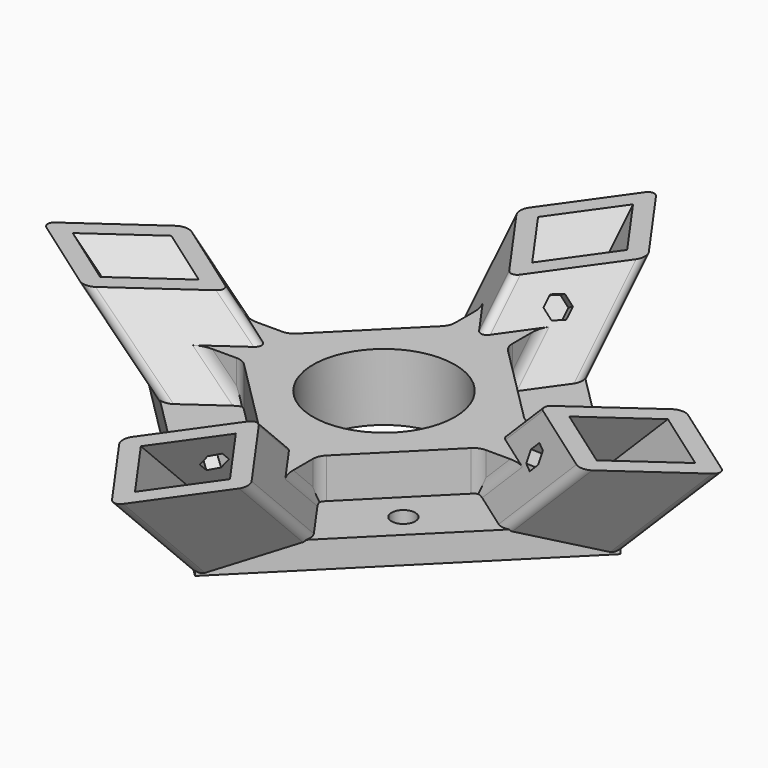
from build123d import *

# Parameters (mm, degrees)
F1_DEPTH      = 4.318
F9_DEPTH      = 2.54
F10_COUNT     = 4
F10_ANGLE     = 270
F14_DEPTH     = 10.795
F12_R         = 11.43
F15_DEPTH     = 25.4
F16_R         = 1.905
F17_DEPTH     = 25.4
F25_W         = 111.76
F25_H         = 15.24
F26_DEPTH     = 152.4
F27_T4_DEPTH  = 14.9351248517
F27_T9_DEPTH  = 24.0949860952
F27_T14_DEPTH = 24.0949860952
F27_T19_DEPTH = 30.2015602576
F27_T24_DEPTH = 30.2015602576
F27_T29_DEPTH = 24.0949860952
F27_T34_DEPTH = 24.0949860952
F27_T39_DEPTH = 24.0949860952
F27_T44_DEPTH = 24.0949860952
F27_T49_DEPTH = 30.2015602576
F27_T54_DEPTH = 30.2015602576
F27_T59_DEPTH = 24.0949860952
F27_T64_DEPTH = 24.0949860952
F27_T69_DEPTH = 14.9351248517
F28_T4_DEPTH  = 24.0949860952
F28_T9_DEPTH  = 24.0949860952
F28_T14_DEPTH = 30.2015602576
F28_T19_DEPTH = 30.2015602576
F28_T24_DEPTH = 24.0949860952
F28_T29_DEPTH = 24.0949860952
F28_T34_DEPTH = 14.9351248517
F28_T39_DEPTH = 14.9351248517
F28_T44_DEPTH = 24.0949860952
F28_T49_DEPTH = 24.0949860952
F28_T54_DEPTH = 24.0949860952
F28_T59_DEPTH = 24.0949860952
F28_T64_DEPTH = 30.2015602576
F28_T69_DEPTH = 30.2015602576
F29_T1_DEPTH  = 9.1072561211
F29_T6_DEPTH  = 14.4203734856
F29_T11_DEPTH = 14.4203734854
F29_T16_DEPTH = 14.4203734856
F29_T21_DEPTH = 14.4203734854
F29_T26_DEPTH = 14.4203734856
F29_T31_DEPTH = 14.4203734854
F29_T36_DEPTH = 14.4203734854
F29_T41_DEPTH = 14.4203734856


# Not quite as in the source:
# - a fillet or chamfer that OpenCascade refuses, or shapes differently, is made with other operations: its cross-section is extruded or revolved along the edge and cut away or added


with BuildPart() as f1:
    # F0 (on Top) → F1 (new body)
    with BuildSketch(Plane.XY):
        Polygon((38.1, 0), (0, 38.1), (-38.1, 0), (0, -38.1), align=None)
    extrude(amount=F1_DEPTH)

    # F5 (on offset) → F6 (join, up to the next surface of F1)
    with BuildSketch(Plane(origin=(0, -35.9210244843, 35.9210244843), x_dir=(1, 0, 0), z_dir=(0, 0.7071067812, -0.7071067812))):
        Polygon((10.5607811984, 16.3799871648), (0, 26.9407683632), (-10.5607811984, 16.3799871648), (0, 5.8192059665), align=None)
        Polygon((-7.1842048969, 16.3799871648), (0, 23.5641920617), (7.1842048969, 16.3799871648), (0, 9.195782268), align=None, mode=Mode.SUBTRACT)
    extrude(until=Until.NEXT)

    # F8 (on offset) → F9 (cut)
    with BuildSketch(Plane(origin=(2.9096029833, -2.0574, -2.0574), x_dir=(-0.4082482905, -0.8660254038, 0.2886751346), z_dir=(-0.7071067812, 0.5, 0.5))):
        Polygon((30.7118833173, 5.5090421757), (32.268461045, 6.6097088424), (32.0935446144, 8.5080780308), (30.3620504561, 9.3057805526), (28.8054727285, 8.2051138859), (28.9803891591, 6.3067446975), align=None)
    extrude(amount=-F9_DEPTH, mode=Mode.SUBTRACT)


with BuildPart() as f10_1:
    # F10: instance of F1
    add(f1.part.rotate(Axis((0, 0, 13.9133725866), (0, 0, 1)), 1 * F10_ANGLE / (F10_COUNT - 1)))


with BuildPart() as f10_2:
    # F10: instance of F1
    add(f1.part.rotate(Axis((0, 0, 13.9133725866), (0, 0, 1)), 2 * F10_ANGLE / (F10_COUNT - 1)))


with BuildPart() as f10_3:
    # F10: instance of F1
    add(f1.part.rotate(Axis((0, 0, 13.9133725866), (0, 0, 1)), 3 * F10_ANGLE / (F10_COUNT - 1)))


with BuildPart() as f1_1:
    add(f1.part)

    add(f10_1.part)  # F14 merges F10_1

    add(f10_2.part)  # F14 merges F10_2

    add(f10_3.part)  # F14 merges F10_3
    # F13 (on Top) → F14 (join)
    with BuildSketch(Plane.XY):
        Polygon((19.05, 4.597891134), (4.5978911339, 19.05), (-4.5978911339, 19.05), (-19.05, 4.5978911339), (-19.05, -4.597891134), (-4.5978911339, -19.05), (4.597891134, -19.05), (19.05, -4.5978911339), align=None)
    extrude(amount=F14_DEPTH)

    # F12 (on offset) → F15 (cut)
    with BuildSketch(Plane.XY.offset(25.4)):
        Circle(F12_R)
    extrude(amount=-F15_DEPTH, mode=Mode.SUBTRACT)

    # F16 (on offset) → F17 (cut)
    with BuildSketch(Plane.XY.offset(25.4)):
        with Locations((-15.6256456507, 15.6256456507)):
            Circle(F16_R)
        with Locations((15.6256456507, 15.6256456507)):
            Circle(F16_R)
        with Locations((15.6256456507, -15.6256456507)):
            Circle(F16_R)
        with Locations((-15.6256456507, -15.6256456507)):
            Circle(F16_R)
    extrude(amount=-F17_DEPTH, mode=Mode.SUBTRACT)

    # F18: union 

    # F19: union 

    # F19_face (on face) → F20 (join, up to the next surface of F1)
    with BuildSketch(Plane(origin=(-19.05, 3.0712475933, 8.6360000001), x_dir=(0, -1, 0), z_dir=(-1, 0, 0))):
        Polygon((3.0532870811, 2.1589999999), (-1.5266435405, 2.1589999999), (-1.5266435405, -4.3180000001), align=None)
        Polygon((7.6691387273, -4.3180000001), (7.6691387273, 2.1589999999), (3.0892081056, 2.1589999999), align=None)
    extrude(until=Until.NEXT)

    # F18_face (on face) → F21 (join, up to the next surface of F1)
    with BuildSketch(Plane(origin=(-3.0712475934, 19.05, 8.636), x_dir=(-1, 0, 0), z_dir=(0, 1, 0))):
        Polygon((1.5266435406, -4.318), (1.5266435406, 2.159), (-3.0532870811, 2.159), align=None)
        Polygon((-3.0892081056, 2.159), (-7.6691387273, 2.159), (-7.6691387273, -4.318), align=None)
    extrude(until=Until.NEXT)

    # F19_face1 (on face) → F22 (join, up to the next surface of F1)
    with BuildSketch(Plane(origin=(19.05, -3.0712475933, 8.6360000001), x_dir=(0, 1, 0), z_dir=(1, 0, 0))):
        Polygon((3.0532870811, 2.1589999999), (-1.5266435405, 2.1589999999), (-1.5266435405, -4.3180000001), align=None)
        Polygon((7.6691387273, -4.3180000001), (7.6691387273, 2.1589999999), (3.0892081056, 2.1589999999), align=None)
    extrude(until=Until.NEXT)

    # F19_face2 (on face) → F23 (join, up to the next surface of F1)
    with BuildSketch(Plane(origin=(3.0712475934, -19.05, 8.636), x_dir=(1, 0, 0), z_dir=(0, -1, 0))):
        Polygon((1.5266435406, -4.318), (1.5266435406, 2.159), (-3.0532870811, 2.159), align=None)
        Polygon((-7.6691387273, -4.3179999998), (-3.0892081056, 2.159), (-7.6691387273, 2.159), align=None)
    extrude(until=Until.NEXT)

    # F25 (on offset) → F26 (cut)
    with BuildSketch(Plane.YZ.offset(63.5)):
        with Locations((0, 24.4856)):
            Rectangle(F25_W, F25_H)
    extrude(amount=-F26_DEPTH, mode=Mode.SUBTRACT)

    # F27: fillet of radius 1.27 on 8 edges, made by hand


with BuildPart() as f27_tool2:
    # F27_s3 → F27_t4 (new body)
    with BuildSketch(Plane(origin=(0, 23.2254640303, 23.2254640303), x_dir=(1, 0, 0), z_dir=(0, -0.7071067812, -0.7071067812))):
        with BuildLine():
            ThreePointArc((0.8980256121, -6.7172315786), (0, -6.3452571907), (-0.8980256121, -6.7172315786))
            Line((-0.8980256121, -6.7172315786), (0, -5.8192059665))
            Line((0, -5.8192059665), (0.8980256121, -6.7172315786))
        make_face()
    extrude(amount=F27_T4_DEPTH)

    split(bisect_by=Plane.XY.offset(10.795), keep=Keep.TOP)


with BuildPart() as f1_2:
    add(f1_1.part)

    # F27_t1: cut F27_tool2
    add(f27_tool2.part, mode=Mode.SUBTRACT)


with BuildPart() as f27_tool7:
    # F27_s8 → F27_t9 (new body)
    with BuildSketch(Plane(origin=(0, 30.6930640303, 30.6930640303), x_dir=(1, 0, 0), z_dir=(0, -0.7071067812, -0.7071067812))):
        with BuildLine():
            ThreePointArc((9.6627555863, -17.2780127769), (10.0347299742, -16.3799871648), (9.6627555863, -15.4819615527))
            Line((9.6627555863, -15.4819615527), (10.5607811984, -16.3799871648))
            Line((10.5607811984, -16.3799871648), (9.6627555863, -17.2780127769))
        make_face()
    extrude(amount=F27_T9_DEPTH)

    split(bisect_by=Plane.XY.offset(4.318), keep=Keep.TOP)


with BuildPart() as f1_3:
    add(f1_2.part)

    # F27_t6: cut F27_tool7
    add(f27_tool7.part, mode=Mode.SUBTRACT)


with BuildPart() as f27_tool12:
    # F27_s13 → F27_t14 (new body)
    with BuildSketch(Plane(origin=(0, 30.6930640303, 30.6930640303), x_dir=(1, 0, 0), z_dir=(0, -0.7071067812, -0.7071067812))):
        with BuildLine():
            ThreePointArc((9.6627555863, -17.2780127769), (10.0347299742, -16.3799871648), (9.6627555863, -15.4819615527))
            Line((9.6627555863, -15.4819615527), (10.5607811984, -16.3799871648))
            Line((10.5607811984, -16.3799871648), (9.6627555863, -17.2780127769))
        make_face()
    extrude(amount=F27_T14_DEPTH)

    split(bisect_by=Plane(origin=(19.05, 19.05, 0), x_dir=(0, 0, 1), z_dir=(0.7071067812, 0.7071067812, 0)), keep=Keep.TOP)


with BuildPart() as f1_4:
    add(f1_3.part)

    # F27_t11: cut F27_tool12
    add(f27_tool12.part, mode=Mode.SUBTRACT)


with BuildPart() as f27_tool17:
    # F27_s18 → F27_t19 (new body)
    with BuildSketch(Plane(origin=(0, 38.1606640303, 38.1606640303), x_dir=(1, 0, 0), z_dir=(0, -0.7071067812, -0.7071067812))):
        with BuildLine():
            ThreePointArc((0.8980256121, -26.0427427511), (0, -26.414717139), (-0.8980256121, -26.0427427511))
            Line((-0.8980256121, -26.0427427511), (0, -26.9407683632))
            Line((0, -26.9407683632), (0.8980256121, -26.0427427511))
        make_face()
    extrude(amount=F27_T19_DEPTH)

    split(bisect_by=Plane(origin=(-19.05, 19.05, 0), x_dir=(0, 0, 1), z_dir=(-0.7071067812, 0.7071067812, 0)), keep=Keep.TOP)


with BuildPart() as f1_5:
    add(f1_4.part)

    # F27_t16: cut F27_tool17
    add(f27_tool17.part, mode=Mode.SUBTRACT)


with BuildPart() as f27_tool22:
    # F27_s23 → F27_t24 (new body)
    with BuildSketch(Plane(origin=(0, 38.1606640303, 38.1606640303), x_dir=(1, 0, 0), z_dir=(0, -0.7071067812, -0.7071067812))):
        with BuildLine():
            ThreePointArc((0.8980256121, -26.0427427511), (0, -26.414717139), (-0.8980256121, -26.0427427511))
            Line((-0.8980256121, -26.0427427511), (0, -26.9407683632))
            Line((0, -26.9407683632), (0.8980256121, -26.0427427511))
        make_face()
    extrude(amount=F27_T24_DEPTH)

    split(bisect_by=Plane(origin=(19.05, 19.05, 0), x_dir=(0, 0, 1), z_dir=(0.7071067812, 0.7071067812, 0)), keep=Keep.TOP)


with BuildPart() as f1_6:
    add(f1_5.part)

    # F27_t21: cut F27_tool22
    add(f27_tool22.part, mode=Mode.SUBTRACT)


with BuildPart() as f27_tool27:
    # F27_s28 → F27_t29 (new body)
    with BuildSketch(Plane(origin=(0, 30.6930640303, 30.6930640303), x_dir=(1, 0, 0), z_dir=(0, -0.7071067812, -0.7071067812))):
        with BuildLine():
            ThreePointArc((-9.6627555863, -17.2780127769), (-10.0347299742, -16.3799871648), (-9.6627555863, -15.4819615527))
            Line((-9.6627555863, -15.4819615527), (-10.5607811984, -16.3799871648))
            Line((-10.5607811984, -16.3799871648), (-9.6627555863, -17.2780127769))
        make_face()
    extrude(amount=F27_T29_DEPTH)

    split(bisect_by=Plane.XY.offset(4.318), keep=Keep.TOP)


with BuildPart() as f1_7:
    add(f1_6.part)

    # F27_t26: cut F27_tool27
    add(f27_tool27.part, mode=Mode.SUBTRACT)


with BuildPart() as f27_tool32:
    # F27_s33 → F27_t34 (new body)
    with BuildSketch(Plane(origin=(0, 30.6930640303, 30.6930640303), x_dir=(1, 0, 0), z_dir=(0, -0.7071067812, -0.7071067812))):
        with BuildLine():
            ThreePointArc((-9.6627555863, -17.2780127769), (-10.0347299742, -16.3799871648), (-9.6627555863, -15.4819615527))
            Line((-9.6627555863, -15.4819615527), (-10.5607811984, -16.3799871648))
            Line((-10.5607811984, -16.3799871648), (-9.6627555863, -17.2780127769))
        make_face()
    extrude(amount=F27_T34_DEPTH)

    split(bisect_by=Plane(origin=(-19.05, 19.05, 0), x_dir=(0, 0, 1), z_dir=(-0.7071067812, 0.7071067812, 0)), keep=Keep.TOP)


with BuildPart() as f1_8:
    add(f1_7.part)

    # F27_t31: cut F27_tool32
    add(f27_tool32.part, mode=Mode.SUBTRACT)


with BuildPart() as f27_tool37:
    # F27_s38 → F27_t39 (new body)
    with BuildSketch(Plane(origin=(30.6930640303, 0, 30.6930640303), x_dir=(0, 1, 0), z_dir=(-0.7071067812, 0, -0.7071067812))):
        with BuildLine():
            ThreePointArc((9.6627555863, 17.2780127769), (10.0347299742, 16.3799871648), (9.6627555863, 15.4819615527))
            Line((9.6627555863, 15.4819615527), (10.5607811984, 16.3799871648))
            Line((10.5607811984, 16.3799871648), (9.6627555863, 17.2780127769))
        make_face()
    extrude(amount=F27_T39_DEPTH)

    split(bisect_by=Plane.XY.offset(4.318), keep=Keep.TOP)


with BuildPart() as f1_9:
    add(f1_8.part)

    # F27_t36: cut F27_tool37
    add(f27_tool37.part, mode=Mode.SUBTRACT)


with BuildPart() as f27_tool42:
    # F27_s43 → F27_t44 (new body)
    with BuildSketch(Plane(origin=(30.6930640303, 0, 30.6930640303), x_dir=(0, 1, 0), z_dir=(-0.7071067812, 0, -0.7071067812))):
        with BuildLine():
            ThreePointArc((9.6627555863, 17.2780127769), (10.0347299742, 16.3799871648), (9.6627555863, 15.4819615527))
            Line((9.6627555863, 15.4819615527), (10.5607811984, 16.3799871648))
            Line((10.5607811984, 16.3799871648), (9.6627555863, 17.2780127769))
        make_face()
    extrude(amount=F27_T44_DEPTH)

    split(bisect_by=Plane(origin=(19.05, 19.05, 0), x_dir=(0, 0, 1), z_dir=(0.7071067812, 0.7071067812, 0)), keep=Keep.TOP)


with BuildPart() as f1_10:
    add(f1_9.part)

    # F27_t41: cut F27_tool42
    add(f27_tool42.part, mode=Mode.SUBTRACT)


with BuildPart() as f27_tool47:
    # F27_s48 → F27_t49 (new body)
    with BuildSketch(Plane(origin=(38.1606640303, 0, 38.1606640303), x_dir=(0, 1, 0), z_dir=(-0.7071067812, 0, -0.7071067812))):
        with BuildLine():
            ThreePointArc((-0.8980256121, 26.0427427511), (0, 26.414717139), (0.8980256121, 26.0427427511))
            Line((0.8980256121, 26.0427427511), (0, 26.9407683632))
            Line((0, 26.9407683632), (-0.8980256121, 26.0427427511))
        make_face()
    extrude(amount=F27_T49_DEPTH)

    split(bisect_by=Plane(origin=(19.05, 19.05, 0), x_dir=(0, 0, 1), z_dir=(0.7071067812, 0.7071067812, 0)), keep=Keep.TOP)


with BuildPart() as f1_11:
    add(f1_10.part)

    # F27_t46: cut F27_tool47
    add(f27_tool47.part, mode=Mode.SUBTRACT)


with BuildPart() as f27_tool52:
    # F27_s53 → F27_t54 (new body)
    with BuildSketch(Plane(origin=(38.1606640303, 0, 38.1606640303), x_dir=(0, 1, 0), z_dir=(-0.7071067812, 0, -0.7071067812))):
        with BuildLine():
            ThreePointArc((-0.8980256121, 26.0427427511), (0, 26.414717139), (0.8980256121, 26.0427427511))
            Line((0.8980256121, 26.0427427511), (0, 26.9407683632))
            Line((0, 26.9407683632), (-0.8980256121, 26.0427427511))
        make_face()
    extrude(amount=F27_T54_DEPTH)

    split(bisect_by=Plane(origin=(19.05, -19.05, 0), x_dir=(0, 0, 1), z_dir=(0.7071067812, -0.7071067812, 0)), keep=Keep.TOP)


with BuildPart() as f1_12:
    add(f1_11.part)

    # F27_t51: cut F27_tool52
    add(f27_tool52.part, mode=Mode.SUBTRACT)


with BuildPart() as f27_tool57:
    # F27_s58 → F27_t59 (new body)
    with BuildSketch(Plane(origin=(30.6930640303, 0, 30.6930640303), x_dir=(0, 1, 0), z_dir=(-0.7071067812, 0, -0.7071067812))):
        with BuildLine():
            ThreePointArc((-9.6627555863, 17.2780127769), (-10.0347299742, 16.3799871648), (-9.6627555863, 15.4819615527))
            Line((-9.6627555863, 15.4819615527), (-10.5607811984, 16.3799871648))
            Line((-10.5607811984, 16.3799871648), (-9.6627555863, 17.2780127769))
        make_face()
    extrude(amount=F27_T59_DEPTH)

    split(bisect_by=Plane.XY.offset(4.318), keep=Keep.TOP)


with BuildPart() as f1_13:
    add(f1_12.part)

    # F27_t56: cut F27_tool57
    add(f27_tool57.part, mode=Mode.SUBTRACT)


with BuildPart() as f27_tool62:
    # F27_s63 → F27_t64 (new body)
    with BuildSketch(Plane(origin=(30.6930640303, 0, 30.6930640303), x_dir=(0, 1, 0), z_dir=(-0.7071067812, 0, -0.7071067812))):
        with BuildLine():
            ThreePointArc((-9.6627555863, 17.2780127769), (-10.0347299742, 16.3799871648), (-9.6627555863, 15.4819615527))
            Line((-9.6627555863, 15.4819615527), (-10.5607811984, 16.3799871648))
            Line((-10.5607811984, 16.3799871648), (-9.6627555863, 17.2780127769))
        make_face()
    extrude(amount=F27_T64_DEPTH)

    split(bisect_by=Plane(origin=(19.05, -19.05, 0), x_dir=(0, 0, 1), z_dir=(0.7071067812, -0.7071067812, 0)), keep=Keep.TOP)


with BuildPart() as f1_14:
    add(f1_13.part)

    # F27_t61: cut F27_tool62
    add(f27_tool62.part, mode=Mode.SUBTRACT)


with BuildPart() as f27_tool67:
    # F27_s68 → F27_t69 (new body)
    with BuildSketch(Plane(origin=(23.2254640303, 0, 23.2254640303), x_dir=(0, 1, 0), z_dir=(-0.7071067812, 0, -0.7071067812))):
        with BuildLine():
            ThreePointArc((-0.8980256121, 6.7172315786), (0, 6.3452571907), (0.8980256121, 6.7172315786))
            Line((0.8980256121, 6.7172315786), (0, 5.8192059665))
            Line((0, 5.8192059665), (-0.8980256121, 6.7172315786))
        make_face()
    extrude(amount=F27_T69_DEPTH)

    split(bisect_by=Plane.XY.offset(10.795), keep=Keep.TOP)


with BuildPart() as f1_15:
    add(f1_14.part)

    # F27_t66: cut F27_tool67
    add(f27_tool67.part, mode=Mode.SUBTRACT)

    # F28: fillet of radius 1.27 on 8 edges, made by hand


with BuildPart() as f28_tool2:
    # F28_s3 → F28_t4 (new body)
    with BuildSketch(Plane(origin=(0, -30.6930640303, 30.6930640303), x_dir=(1, 0, 0), z_dir=(0, 0.7071067812, -0.7071067812))):
        with BuildLine():
            ThreePointArc((-9.6627555863, 17.2780127769), (-10.0347299742, 16.3799871648), (-9.6627555863, 15.4819615527))
            Line((-9.6627555863, 15.4819615527), (-10.5607811984, 16.3799871648))
            Line((-10.5607811984, 16.3799871648), (-9.6627555863, 17.2780127769))
        make_face()
    extrude(amount=F28_T4_DEPTH)

    split(bisect_by=Plane.XY.offset(4.318), keep=Keep.TOP)


with BuildPart() as f1_16:
    add(f1_15.part)

    # F28_t1: cut F28_tool2
    add(f28_tool2.part, mode=Mode.SUBTRACT)


with BuildPart() as f28_tool7:
    # F28_s8 → F28_t9 (new body)
    with BuildSketch(Plane(origin=(0, -30.6930640303, 30.6930640303), x_dir=(1, 0, 0), z_dir=(0, 0.7071067812, -0.7071067812))):
        with BuildLine():
            ThreePointArc((-9.6627555863, 17.2780127769), (-10.0347299742, 16.3799871648), (-9.6627555863, 15.4819615527))
            Line((-9.6627555863, 15.4819615527), (-10.5607811984, 16.3799871648))
            Line((-10.5607811984, 16.3799871648), (-9.6627555863, 17.2780127769))
        make_face()
    extrude(amount=F28_T9_DEPTH)

    split(bisect_by=Plane(origin=(-19.05, -19.05, 0), x_dir=(0, 0, 1), z_dir=(-0.7071067812, -0.7071067812, 0)), keep=Keep.TOP)


with BuildPart() as f1_17:
    add(f1_16.part)

    # F28_t6: cut F28_tool7
    add(f28_tool7.part, mode=Mode.SUBTRACT)


with BuildPart() as f28_tool12:
    # F28_s13 → F28_t14 (new body)
    with BuildSketch(Plane(origin=(0, -38.1606640303, 38.1606640303), x_dir=(1, 0, 0), z_dir=(0, 0.7071067812, -0.7071067812))):
        with BuildLine():
            ThreePointArc((0.8980256121, 26.0427427511), (0, 26.414717139), (-0.8980256121, 26.0427427511))
            Line((-0.8980256121, 26.0427427511), (0, 26.9407683632))
            Line((0, 26.9407683632), (0.8980256121, 26.0427427511))
        make_face()
    extrude(amount=F28_T14_DEPTH)

    split(bisect_by=Plane(origin=(-19.05, -19.05, 0), x_dir=(0, 0, 1), z_dir=(-0.7071067812, -0.7071067812, 0)), keep=Keep.TOP)


with BuildPart() as f1_18:
    add(f1_17.part)

    # F28_t11: cut F28_tool12
    add(f28_tool12.part, mode=Mode.SUBTRACT)


with BuildPart() as f28_tool17:
    # F28_s18 → F28_t19 (new body)
    with BuildSketch(Plane(origin=(0, -38.1606640303, 38.1606640303), x_dir=(1, 0, 0), z_dir=(0, 0.7071067812, -0.7071067812))):
        with BuildLine():
            ThreePointArc((0.8980256121, 26.0427427511), (0, 26.414717139), (-0.8980256121, 26.0427427511))
            Line((-0.8980256121, 26.0427427511), (0, 26.9407683632))
            Line((0, 26.9407683632), (0.8980256121, 26.0427427511))
        make_face()
    extrude(amount=F28_T19_DEPTH)

    split(bisect_by=Plane(origin=(19.05, -19.05, 0), x_dir=(0, 0, 1), z_dir=(0.7071067812, -0.7071067812, 0)), keep=Keep.TOP)


with BuildPart() as f1_19:
    add(f1_18.part)

    # F28_t16: cut F28_tool17
    add(f28_tool17.part, mode=Mode.SUBTRACT)


with BuildPart() as f28_tool22:
    # F28_s23 → F28_t24 (new body)
    with BuildSketch(Plane(origin=(0, -30.6930640303, 30.6930640303), x_dir=(1, 0, 0), z_dir=(0, 0.7071067812, -0.7071067812))):
        with BuildLine():
            ThreePointArc((9.6627555863, 17.2780127769), (10.0347299742, 16.3799871648), (9.6627555863, 15.4819615527))
            Line((9.6627555863, 15.4819615527), (10.5607811984, 16.3799871648))
            Line((10.5607811984, 16.3799871648), (9.6627555863, 17.2780127769))
        make_face()
    extrude(amount=F28_T24_DEPTH)

    split(bisect_by=Plane.XY.offset(4.318), keep=Keep.TOP)


with BuildPart() as f1_20:
    add(f1_19.part)

    # F28_t21: cut F28_tool22
    add(f28_tool22.part, mode=Mode.SUBTRACT)


with BuildPart() as f28_tool27:
    # F28_s28 → F28_t29 (new body)
    with BuildSketch(Plane(origin=(0, -30.6930640303, 30.6930640303), x_dir=(1, 0, 0), z_dir=(0, 0.7071067812, -0.7071067812))):
        with BuildLine():
            ThreePointArc((9.6627555863, 17.2780127769), (10.0347299742, 16.3799871648), (9.6627555863, 15.4819615527))
            Line((9.6627555863, 15.4819615527), (10.5607811984, 16.3799871648))
            Line((10.5607811984, 16.3799871648), (9.6627555863, 17.2780127769))
        make_face()
    extrude(amount=F28_T29_DEPTH)

    split(bisect_by=Plane(origin=(19.05, -19.05, 0), x_dir=(0, 0, 1), z_dir=(0.7071067812, -0.7071067812, 0)), keep=Keep.TOP)


with BuildPart() as f1_21:
    add(f1_20.part)

    # F28_t26: cut F28_tool27
    add(f28_tool27.part, mode=Mode.SUBTRACT)


with BuildPart() as f28_tool32:
    # F28_s33 → F28_t34 (new body)
    with BuildSketch(Plane(origin=(0, -23.2254640303, 23.2254640303), x_dir=(1, 0, 0), z_dir=(0, 0.7071067812, -0.7071067812))):
        with BuildLine():
            ThreePointArc((0.8980256121, 6.7172315786), (0, 6.3452571907), (-0.8980256121, 6.7172315786))
            Line((-0.8980256121, 6.7172315786), (0, 5.8192059665))
            Line((0, 5.8192059665), (0.8980256121, 6.7172315786))
        make_face()
    extrude(amount=F28_T34_DEPTH)

    split(bisect_by=Plane.XY.offset(10.795), keep=Keep.TOP)


with BuildPart() as f1_22:
    add(f1_21.part)

    # F28_t31: cut F28_tool32
    add(f28_tool32.part, mode=Mode.SUBTRACT)


with BuildPart() as f28_tool37:
    # F28_s38 → F28_t39 (new body)
    with BuildSketch(Plane(origin=(-23.2254640303, 0, 23.2254640303), x_dir=(0, 1, 0), z_dir=(0.7071067812, 0, -0.7071067812))):
        with BuildLine():
            ThreePointArc((-0.8980256121, -6.7172315786), (0, -6.3452571907), (0.8980256121, -6.7172315786))
            Line((0.8980256121, -6.7172315786), (0, -5.8192059665))
            Line((0, -5.8192059665), (-0.8980256121, -6.7172315786))
        make_face()
    extrude(amount=F28_T39_DEPTH)

    split(bisect_by=Plane.XY.offset(10.795), keep=Keep.TOP)


with BuildPart() as f1_23:
    add(f1_22.part)

    # F28_t36: cut F28_tool37
    add(f28_tool37.part, mode=Mode.SUBTRACT)


with BuildPart() as f28_tool42:
    # F28_s43 → F28_t44 (new body)
    with BuildSketch(Plane(origin=(-30.6930640303, 0, 30.6930640303), x_dir=(0, 1, 0), z_dir=(0.7071067812, 0, -0.7071067812))):
        with BuildLine():
            ThreePointArc((-9.6627555863, -17.2780127769), (-10.0347299742, -16.3799871648), (-9.6627555863, -15.4819615527))
            Line((-9.6627555863, -15.4819615527), (-10.5607811984, -16.3799871648))
            Line((-10.5607811984, -16.3799871648), (-9.6627555863, -17.2780127769))
        make_face()
    extrude(amount=F28_T44_DEPTH)

    split(bisect_by=Plane.XY.offset(4.318), keep=Keep.TOP)


with BuildPart() as f1_24:
    add(f1_23.part)

    # F28_t41: cut F28_tool42
    add(f28_tool42.part, mode=Mode.SUBTRACT)


with BuildPart() as f28_tool47:
    # F28_s48 → F28_t49 (new body)
    with BuildSketch(Plane(origin=(-30.6930640303, 0, 30.6930640303), x_dir=(0, 1, 0), z_dir=(0.7071067812, 0, -0.7071067812))):
        with BuildLine():
            ThreePointArc((-9.6627555863, -17.2780127769), (-10.0347299742, -16.3799871648), (-9.6627555863, -15.4819615527))
            Line((-9.6627555863, -15.4819615527), (-10.5607811984, -16.3799871648))
            Line((-10.5607811984, -16.3799871648), (-9.6627555863, -17.2780127769))
        make_face()
    extrude(amount=F28_T49_DEPTH)

    split(bisect_by=Plane(origin=(-19.05, -19.05, 0), x_dir=(0, 0, 1), z_dir=(-0.7071067812, -0.7071067812, 0)), keep=Keep.TOP)


with BuildPart() as f1_25:
    add(f1_24.part)

    # F28_t46: cut F28_tool47
    add(f28_tool47.part, mode=Mode.SUBTRACT)


with BuildPart() as f28_tool52:
    # F28_s53 → F28_t54 (new body)
    with BuildSketch(Plane(origin=(-30.6930640303, 0, 30.6930640303), x_dir=(0, 1, 0), z_dir=(0.7071067812, 0, -0.7071067812))):
        with BuildLine():
            ThreePointArc((9.6627555863, -17.2780127769), (10.0347299742, -16.3799871648), (9.6627555863, -15.4819615527))
            Line((9.6627555863, -15.4819615527), (10.5607811984, -16.3799871648))
            Line((10.5607811984, -16.3799871648), (9.6627555863, -17.2780127769))
        make_face()
    extrude(amount=F28_T54_DEPTH)

    split(bisect_by=Plane.XY.offset(4.318), keep=Keep.TOP)


with BuildPart() as f1_26:
    add(f1_25.part)

    # F28_t51: cut F28_tool52
    add(f28_tool52.part, mode=Mode.SUBTRACT)


with BuildPart() as f28_tool57:
    # F28_s58 → F28_t59 (new body)
    with BuildSketch(Plane(origin=(-30.6930640303, 0, 30.6930640303), x_dir=(0, 1, 0), z_dir=(0.7071067812, 0, -0.7071067812))):
        with BuildLine():
            ThreePointArc((9.6627555863, -17.2780127769), (10.0347299742, -16.3799871648), (9.6627555863, -15.4819615527))
            Line((9.6627555863, -15.4819615527), (10.5607811984, -16.3799871648))
            Line((10.5607811984, -16.3799871648), (9.6627555863, -17.2780127769))
        make_face()
    extrude(amount=F28_T59_DEPTH)

    split(bisect_by=Plane(origin=(-19.05, 19.05, 0), x_dir=(0, 0, 1), z_dir=(-0.7071067812, 0.7071067812, 0)), keep=Keep.TOP)


with BuildPart() as f1_27:
    add(f1_26.part)

    # F28_t56: cut F28_tool57
    add(f28_tool57.part, mode=Mode.SUBTRACT)


with BuildPart() as f28_tool62:
    # F28_s63 → F28_t64 (new body)
    with BuildSketch(Plane(origin=(-38.1606640303, 0, 38.1606640303), x_dir=(0, 1, 0), z_dir=(0.7071067812, 0, -0.7071067812))):
        with BuildLine():
            ThreePointArc((-0.8980256121, -26.0427427511), (0, -26.414717139), (0.8980256121, -26.0427427511))
            Line((0.8980256121, -26.0427427511), (0, -26.9407683632))
            Line((0, -26.9407683632), (-0.8980256121, -26.0427427511))
        make_face()
    extrude(amount=F28_T64_DEPTH)

    split(bisect_by=Plane(origin=(-19.05, 19.05, 0), x_dir=(0, 0, 1), z_dir=(-0.7071067812, 0.7071067812, 0)), keep=Keep.TOP)


with BuildPart() as f1_28:
    add(f1_27.part)

    # F28_t61: cut F28_tool62
    add(f28_tool62.part, mode=Mode.SUBTRACT)


with BuildPart() as f28_tool67:
    # F28_s68 → F28_t69 (new body)
    with BuildSketch(Plane(origin=(-38.1606640303, 0, 38.1606640303), x_dir=(0, 1, 0), z_dir=(0.7071067812, 0, -0.7071067812))):
        with BuildLine():
            ThreePointArc((-0.8980256121, -26.0427427511), (0, -26.414717139), (0.8980256121, -26.0427427511))
            Line((0.8980256121, -26.0427427511), (0, -26.9407683632))
            Line((0, -26.9407683632), (-0.8980256121, -26.0427427511))
        make_face()
    extrude(amount=F28_T69_DEPTH)

    split(bisect_by=Plane(origin=(-19.05, -19.05, 0), x_dir=(0, 0, 1), z_dir=(-0.7071067812, -0.7071067812, 0)), keep=Keep.TOP)


with BuildPart() as f1_29:
    add(f1_28.part)

    # F28_t66: cut F28_tool67
    add(f28_tool67.part, mode=Mode.SUBTRACT)

    # F29: fillet of radius 2.54 on 16 edges, made by hand

    # F29_s2 → F29_t1 (join)
    with BuildSketch(Plane.XY.offset(1.6877438789)):
        with BuildLine():
            ThreePointArc((18.3060512242, 5.3418399098), (19.1300865302, 4.7912371214), (20.1021024484, 4.597891134))
            Line((20.1021024484, 4.597891134), (19.05, 4.597891134))
            Line((19.05, 4.597891134), (18.3060512242, 5.3418399098))
        make_face()
        with BuildLine():
            ThreePointArc((4.5978911339, 20.1021024484), (4.7912371213, 19.1300865302), (5.3418399097, 18.3060512242))
            Line((5.3418399097, 18.3060512242), (4.5978911339, 19.05))
            Line((4.5978911339, 19.05), (4.5978911339, 20.1021024484))
        make_face()
        with BuildLine():
            ThreePointArc((-5.3418399097, 18.3060512242), (-4.7912371213, 19.1300865302), (-4.5978911339, 20.1021024484))
            Line((-4.5978911339, 20.1021024484), (-4.5978911339, 19.05))
            Line((-4.5978911339, 19.05), (-5.3418399097, 18.3060512242))
        make_face()
        with BuildLine():
            ThreePointArc((-20.1021024484, 4.5978911339), (-19.1300865302, 4.7912371213), (-18.3060512242, 5.3418399097))
            Line((-18.3060512242, 5.3418399097), (-19.05, 4.5978911339))
            Line((-19.05, 4.5978911339), (-20.1021024484, 4.5978911339))
        make_face()
        with BuildLine():
            ThreePointArc((-18.3060512242, -5.3418399097), (-19.1300865302, -4.7912371214), (-20.1021024484, -4.597891134))
            Line((-20.1021024484, -4.597891134), (-19.05, -4.597891134))
            Line((-19.05, -4.597891134), (-18.3060512242, -5.3418399097))
        make_face()
        with BuildLine():
            ThreePointArc((-4.5978911339, -20.1021024484), (-4.7912371213, -19.1300865302), (-5.3418399097, -18.3060512242))
            Line((-5.3418399097, -18.3060512242), (-4.5978911339, -19.05))
            Line((-4.5978911339, -19.05), (-4.5978911339, -20.1021024484))
        make_face()
        with BuildLine():
            ThreePointArc((5.3418399097, -18.3060512242), (4.7912371214, -19.1300865302), (4.597891134, -20.1021024484))
            Line((4.597891134, -20.1021024484), (4.597891134, -19.05))
            Line((4.597891134, -19.05), (5.3418399097, -18.3060512242))
        make_face()
        with BuildLine():
            ThreePointArc((20.1021024484, -4.5978911339), (19.1300865302, -4.7912371213), (18.3060512242, -5.3418399097))
            Line((18.3060512242, -5.3418399097), (19.05, -4.5978911339))
            Line((19.05, -4.5978911339), (20.1021024484, -4.5978911339))
        make_face()
    extrude(amount=F29_T1_DEPTH)


with BuildPart() as f29_tool4:
    # F29_s5 → F29_t6 (new body)
    with BuildSketch(Plane(origin=(20.0208719395, 0, 20.0208719395), x_dir=(0, 1, 0), z_dir=(-0.7071067812, 0, -0.7071067812))):
        with BuildLine():
            ThreePointArc((5.3418399098, 11.1610458762), (4.7912371214, 10.3370105702), (4.597891134, 9.364994652))
            Line((4.597891134, 9.364994652), (4.597891134, 10.4170971004))
            Line((4.597891134, 10.4170971004), (5.3418399098, 11.1610458762))
        make_face()
    extrude(amount=F29_T6_DEPTH)

    split(bisect_by=Plane.XY.offset(10.795), keep=Keep.BOTTOM)


with BuildPart() as f1_30:
    add(f1_29.part)

    # F29_t3: union F29_tool4
    add(f29_tool4.part)


with BuildPart() as f29_tool9:
    # F29_s10 → F29_t11 (new body)
    with BuildSketch(Plane(origin=(0, -9.8241280606, 9.8241280606), x_dir=(1, 0, 0), z_dir=(0, -0.7071067812, 0.7071067812))):
        with BuildLine():
            ThreePointArc((-5.3418399097, -11.1610458761), (-4.7912371213, -10.3370105701), (-4.5978911339, -9.3649946519))
            Line((-4.5978911339, -9.3649946519), (-4.5978911339, -10.4170971004))
            Line((-4.5978911339, -10.4170971004), (-5.3418399097, -11.1610458761))
        make_face()
    extrude(amount=F29_T11_DEPTH)

    split(bisect_by=Plane.XY.offset(10.795), keep=Keep.BOTTOM)


with BuildPart() as f1_31:
    add(f1_30.part)

    # F29_t8: union F29_tool9
    add(f29_tool9.part)


with BuildPart() as f29_tool14:
    # F29_s15 → F29_t16 (new body)
    with BuildSketch(Plane(origin=(-20.0208719394, 0, 20.0208719394), x_dir=(0, 1, 0), z_dir=(0.7071067812, 0, -0.7071067812))):
        with BuildLine():
            ThreePointArc((-4.597891134, -9.364994652), (-4.7912371214, -10.3370105702), (-5.3418399097, -11.1610458762))
            Line((-5.3418399097, -11.1610458762), (-4.597891134, -10.4170971004))
            Line((-4.597891134, -10.4170971004), (-4.597891134, -9.364994652))
        make_face()
    extrude(amount=F29_T16_DEPTH)

    split(bisect_by=Plane.XY.offset(10.795), keep=Keep.BOTTOM)


with BuildPart() as f1_32:
    add(f1_31.part)

    # F29_t13: union F29_tool14
    add(f29_tool14.part)


with BuildPart() as f29_tool19:
    # F29_s20 → F29_t21 (new body)
    with BuildSketch(Plane(origin=(-9.8241280606, 0, 9.8241280606), x_dir=(0, 1, 0), z_dir=(-0.7071067812, 0, 0.7071067812))):
        with BuildLine():
            ThreePointArc((5.3418399097, 11.1610458761), (4.7912371213, 10.3370105701), (4.5978911339, 9.3649946519))
            Line((4.5978911339, 9.3649946519), (4.5978911339, 10.4170971003))
            Line((4.5978911339, 10.4170971003), (5.3418399097, 11.1610458761))
        make_face()
    extrude(amount=F29_T21_DEPTH)

    split(bisect_by=Plane.XY.offset(10.795), keep=Keep.BOTTOM)


with BuildPart() as f1_33:
    add(f1_32.part)

    # F29_t18: union F29_tool19
    add(f29_tool19.part)


with BuildPart() as f29_tool24:
    # F29_s25 → F29_t26 (new body)
    with BuildSketch(Plane(origin=(0, 20.0208719394, 20.0208719394), x_dir=(1, 0, 0), z_dir=(0, -0.7071067812, -0.7071067812))):
        with BuildLine():
            ThreePointArc((-4.5978911339, -9.364994652), (-4.7912371213, -10.3370105702), (-5.3418399097, -11.1610458762))
            Line((-5.3418399097, -11.1610458762), (-4.5978911339, -10.4170971004))
            Line((-4.5978911339, -10.4170971004), (-4.5978911339, -9.364994652))
        make_face()
    extrude(amount=F29_T26_DEPTH)

    split(bisect_by=Plane.XY.offset(10.795), keep=Keep.BOTTOM)


with BuildPart() as f1_34:
    add(f1_33.part)

    # F29_t23: union F29_tool24
    add(f29_tool24.part)


with BuildPart() as f29_tool29:
    # F29_s30 → F29_t31 (new body)
    with BuildSketch(Plane(origin=(0, 9.8241280606, 9.8241280606), x_dir=(1, 0, 0), z_dir=(0, 0.7071067812, 0.7071067812))):
        with BuildLine():
            ThreePointArc((5.3418399097, 11.1610458761), (4.7912371213, 10.3370105701), (4.5978911339, 9.3649946519))
            Line((4.5978911339, 9.3649946519), (4.5978911339, 10.4170971004))
            Line((4.5978911339, 10.4170971004), (5.3418399097, 11.1610458761))
        make_face()
    extrude(amount=F29_T31_DEPTH)

    split(bisect_by=Plane.XY.offset(10.795), keep=Keep.BOTTOM)


with BuildPart() as f1_35:
    add(f1_34.part)

    # F29_t28: union F29_tool29
    add(f29_tool29.part)


with BuildPart() as f29_tool34:
    # F29_s35 → F29_t36 (new body)
    with BuildSketch(Plane(origin=(9.8241280606, 0, 9.8241280606), x_dir=(0, 1, 0), z_dir=(0.7071067812, 0, 0.7071067812))):
        with BuildLine():
            ThreePointArc((-4.5978911339, -9.3649946519), (-4.7912371213, -10.3370105701), (-5.3418399097, -11.1610458761))
            Line((-5.3418399097, -11.1610458761), (-4.5978911339, -10.4170971003))
            Line((-4.5978911339, -10.4170971003), (-4.5978911339, -9.3649946519))
        make_face()
    extrude(amount=F29_T36_DEPTH)

    split(bisect_by=Plane.XY.offset(10.795), keep=Keep.BOTTOM)


with BuildPart() as f1_36:
    add(f1_35.part)

    # F29_t33: union F29_tool34
    add(f29_tool34.part)


with BuildPart() as f29_tool39:
    # F29_s40 → F29_t41 (new body)
    with BuildSketch(Plane(origin=(0, -20.0208719394, 20.0208719394), x_dir=(1, 0, 0), z_dir=(0, 0.7071067812, -0.7071067812))):
        with BuildLine():
            ThreePointArc((4.597891134, 9.364994652), (4.7912371214, 10.3370105702), (5.3418399097, 11.1610458762))
            Line((5.3418399097, 11.1610458762), (4.597891134, 10.4170971004))
            Line((4.597891134, 10.4170971004), (4.597891134, 9.364994652))
        make_face()
    extrude(amount=F29_T41_DEPTH)

    split(bisect_by=Plane.XY.offset(10.795), keep=Keep.BOTTOM)


with BuildPart() as f1_37:
    add(f1_36.part)

    # F29_t38: union F29_tool39
    add(f29_tool39.part)


solid = f1_37.part
